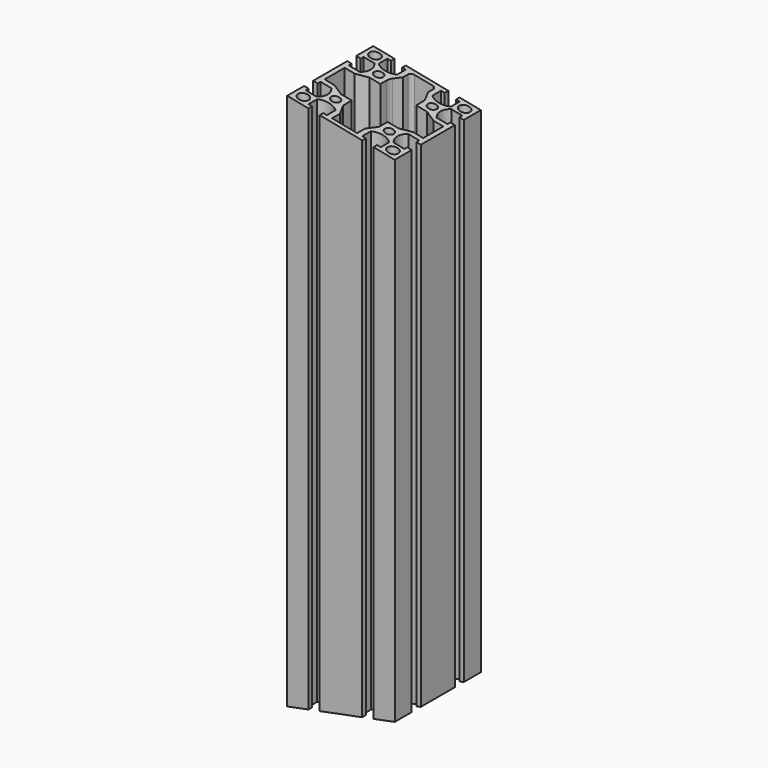
from build123d import *

# Parameters (mm, degrees)
F0_R          = 3
F0_R_2        = 2.5
F1_DEPTH      = 300
F2_R          = 2
F3_R          = 7
F6_DEPTH      = 30
F6_DEPTH_BACK = 30


# Not quite as in the source:
# - a feature names something its author has since deleted; it is built from what else it names


with BuildPart() as f1:
    # F0 (on Top) → F1 (new body)
    with BuildSketch(Plane.XY):
        with BuildLine():
            Line((18.15, -30), (30, -30))
            Line((30, -30), (30, -18.15))
            Line((30, -18.15), (27.5, -18.15))
            Line((27.5, -18.15), (27.5, -20.15))
            Line((27.5, -20.15), (21.5477069044, -20.15))
            ThreePointArc((21.5477069044, -20.15), (19.5, -15), (21.5477069044, -9.85))
            Line((21.5477069044, -9.85), (27.5, -9.85))
            Line((27.5, -9.85), (27.5, -11.85))
            Line((27.5, -11.85), (30, -11.85))
            Line((30, -11.85), (30, 11.85))
            Line((30, 11.85), (27.5, 11.85))
            Line((27.5, 11.85), (27.5, 9.85))
            Line((27.5, 9.85), (21.5477069044, 9.85))
            ThreePointArc((21.5477069044, 9.85), (19.5, 15), (21.5477069044, 20.15))
            Line((21.5477069044, 20.15), (27.5, 20.15))
            Line((27.5, 20.15), (27.5, 18.15))
            Line((27.5, 18.15), (30, 18.15))
            Line((30, 18.15), (30, 30))
            Line((30, 30), (18.15, 30))
            Line((18.15, 30), (18.15, 27.5))
            Line((18.15, 27.5), (20.15, 27.5))
            Line((20.15, 27.5), (20.15, 21.5477069044))
            ThreePointArc((20.15, 21.5477069044), (15, 19.5), (9.85, 21.5477069044))
            Line((9.85, 21.5477069044), (9.85, 27.5))
            Line((9.85, 27.5), (11.85, 27.5))
            Line((11.85, 27.5), (11.85, 30))
            Line((11.85, 30), (-11.85, 30))
            Line((-11.85, 30), (-11.85, 27.5))
            Line((-11.85, 27.5), (-9.85, 27.5))
            Line((-9.85, 27.5), (-9.85, 21.5477069044))
            ThreePointArc((-9.85, 21.5477069044), (-15, 19.5), (-20.15, 21.5477069044))
            Line((-20.15, 21.5477069044), (-20.15, 27.5))
            Line((-20.15, 27.5), (-18.15, 27.5))
            Line((-18.15, 27.5), (-18.15, 30))
            Line((-18.15, 30), (-30, 30))
            Line((-30, 30), (-30, 18.15))
            Line((-30, 18.15), (-27.5, 18.15))
            Line((-27.5, 18.15), (-27.5, 20.15))
            Line((-27.5, 20.15), (-21.5477069044, 20.15))
            ThreePointArc((-21.5477069044, 20.15), (-19.5, 15), (-21.5477069044, 9.85))
            Line((-21.5477069044, 9.85), (-27.5, 9.85))
            Line((-27.5, 9.85), (-27.5, 11.85))
            Line((-27.5, 11.85), (-30, 11.85))
            Line((-30, 11.85), (-30, -11.85))
            Line((-30, -11.85), (-27.5, -11.85))
            Line((-27.5, -11.85), (-27.5, -9.85))
            Line((-27.5, -9.85), (-21.5477069044, -9.85))
            ThreePointArc((-21.5477069044, -9.85), (-19.5, -15), (-21.5477069044, -20.15))
            Line((-21.5477069044, -20.15), (-27.5, -20.15))
            Line((-27.5, -20.15), (-27.5, -18.15))
            Line((-27.5, -18.15), (-30, -18.15))
            Line((-30, -18.15), (-30, -30))
            Line((-30, -30), (-18.15, -30))
            Line((-18.15, -30), (-18.15, -27.5))
            Line((-18.15, -27.5), (-20.15, -27.5))
            Line((-20.15, -27.5), (-20.15, -21.5477069044))
            ThreePointArc((-20.15, -21.5477069044), (-15, -19.5), (-9.85, -21.5477069044))
            Line((-9.85, -21.5477069044), (-9.85, -27.5))
            Line((-9.85, -27.5), (-11.85, -27.5))
            Line((-11.85, -27.5), (-11.85, -30))
            Line((-11.85, -30), (11.85, -30))
            Line((11.85, -30), (11.85, -27.5))
            Line((11.85, -27.5), (9.85, -27.5))
            Line((9.85, -27.5), (9.85, -21.5477069044))
            ThreePointArc((9.85, -21.5477069044), (15, -19.5), (20.15, -21.5477069044))
            Line((20.15, -21.5477069044), (20.15, -27.5))
            Line((20.15, -27.5), (18.15, -27.5))
            Line((18.15, -27.5), (18.15, -30))
        make_face()
        with Locations((-25, -25)):
            Circle(F0_R, mode=Mode.SUBTRACT)
        with Locations((-15, -15)):
            Circle(F0_R_2, mode=Mode.SUBTRACT)
        with Locations((25, -25)):
            Circle(F0_R, mode=Mode.SUBTRACT)
        with Locations((15, -15)):
            Circle(F0_R_2, mode=Mode.SUBTRACT)
        with Locations((-25, 25)):
            Circle(F0_R, mode=Mode.SUBTRACT)
        with Locations((-15, 15)):
            Circle(F0_R_2, mode=Mode.SUBTRACT)
        Polygon((-7, 22), (-7, 27.5), (0, 27.5), (7, 27.5), (7, 22), (10, 16), (10, 10), (16, 10), (22, 7), (27.5, 7), (27.5, 0), (27.5, -7), (22, -7), (16, -10), (10, -10), (10, -16), (7, -22), (7, -27.5), (0, -27.5), (-7, -27.5), (-7, -22), (-10, -16), (-10, -10), (-16, -10), (-22, -7), (-27.5, -7), (-27.5, 0), (-27.5, 7), (-22, 7), (-16, 10), (-10, 10), (-10, 16), align=None, mode=Mode.SUBTRACT)
        with Locations((15, 15)):
            Circle(F0_R_2, mode=Mode.SUBTRACT)
        with Locations((25, 25)):
            Circle(F0_R, mode=Mode.SUBTRACT)
    extrude(amount=F1_DEPTH)

    # F2
    f2_edges = [f1.edges().sort_by_distance(p)[0] for p in [
        (-7, 27.5, 150),
        (7, 27.5, 150),
    ]]
    fillet(f2_edges, radius=F2_R)

    # F3
    f3_edges = [f1.edges().sort_by_distance(p)[0] for p in [
        (-10, 16, 150),
        (10, 16, 150),
    ]]
    fillet(f3_edges, radius=F3_R)

    # F5 (on Front) → F6 (cut, two sides)
    with BuildSketch(Plane.XZ) as f6_sk:
        Polygon((-5.0746062651, -125.30841628), (210.6737913168, -82.3933917586), (185.748397582, 42.9150245214), (-30, 0), align=None)
        Polygon((73.2666294749, 279.4589902598), (110.3184495721, 465.7310686897), (7.0518200972, 486.2720784299), (-30, 300), align=None)
    extrude(amount=F6_DEPTH, mode=Mode.SUBTRACT)
    extrude(f6_sk.sketch, amount=-F6_DEPTH_BACK, mode=Mode.SUBTRACT)


solid = f1.part
